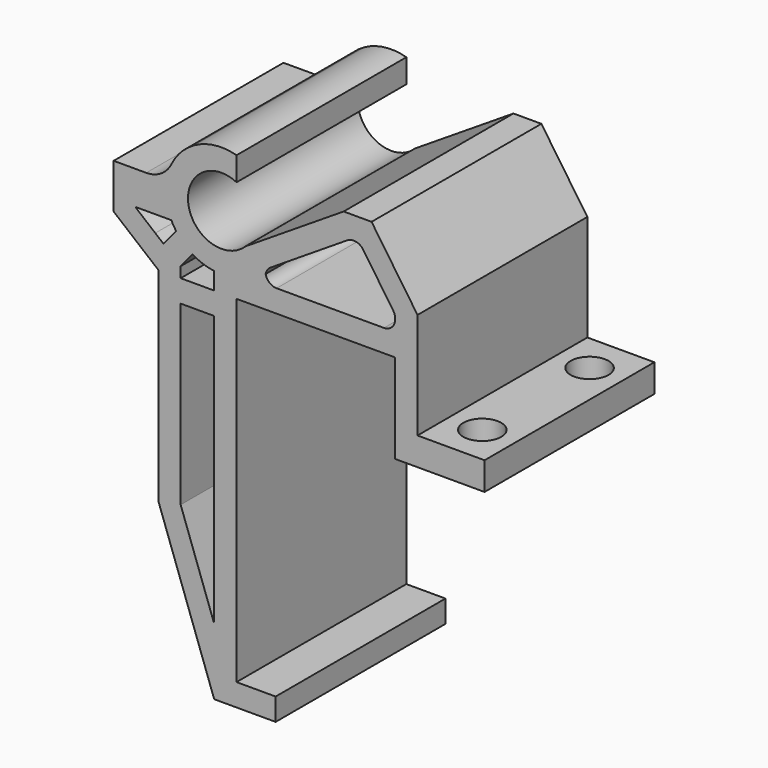
from build123d import *

# Parameters (mm, degrees)
F0_W        = 3
F0_H        = 2
F1_DEPTH    = 19
F3_D        = 3.4
F4_T1_DEPTH = 19


# Not quite as in the source:
# - a fillet or chamfer that OpenCascade refuses, or shapes differently, is made with other operations: its cross-section is extruded or revolved along the edge and cut away or added


with BuildPart() as f1:
    # F0 (on Front) → F1 (new body)
    with BuildSketch(Plane.XZ):
        with Locations((-7, 31.2)):
            Rectangle(F0_W, F0_H)
        with BuildLine():
            Line((-10.0427465571, 34.4155443421), (-8.5, 33.1427784325))
            Line((-8.5, 33.1427784325), (-7.441074238, 34.4263248107))
            ThreePointArc((-7.441074238, 34.4263248107), (-8.244619139, 35.032889635), (-8.9103596286, 35.7881345584))
            Line((-8.9103596286, 35.7881345584), (-10.0427465571, 34.4155443421))
        make_face()
        with BuildLine():
            Line((-10.5, 14), (-5.5, 0))
            Line((-5.5, 0), (-5.5, 5.9464274989))
            Line((-5.5, 5.9464274989), (-8.5, 14.3464274989))
            Line((-8.5, 14.3464274989), (-8.5, 30.2))
            Line((-8.5, 30.2), (-8.5, 32.2))
            Line((-8.5, 32.2), (-8.5, 33.1427784325))
            Line((-8.5, 33.1427784325), (-10.0427465571, 34.4155443421))
            Line((-10.0427465571, 34.4155443421), (-10.7699806475, 35.0155124667))
            Line((-10.7699806475, 35.0155124667), (-12.5, 36.4427784325))
            Line((-12.5, 36.4427784325), (-12.5, 36.5))
            Line((-12.5, 36.5), (-9.3357403136, 36.5))
            ThreePointArc((-9.3357403136, 36.5), (-9.7907115521, 37.9601557031), (-9.7830217401, 39.4895328221))
            ThreePointArc((-9.7830217401, 39.4895328221), (-9.7333018776, 39.7544433664), (-9.6693788597, 40.0162897125))
            ThreePointArc((-9.6693788597, 40.0162897125), (-9.5234750406, 40.4660413374), (-9.3357403136, 40.9))
            ThreePointArc((-9.3357403136, 40.9), (-10.2578590901, 39.8786796564), (-11.5807347457, 39.5))
            Line((-11.5807347457, 39.5), (-14.5, 39.5))
            Line((-14.5, 39.5), (-14.5, 35.5))
            Line((-14.5, 35.5), (-10.5, 32.2))
            Line((-10.5, 32.2), (-10.5, 14))
        make_face()
        with BuildLine():
            Line((-4.3254974298, 0), (0, 0))
            Line((0, 0), (0, 2))
            Line((0, 2), (-3.5, 2))
            Line((-3.5, 2), (-3.5, 32.2))
            Line((-3.5, 32.2), (6, 32.2))
            Line((6, 32.2), (10.7, 32.2))
            Line((10.7, 32.2), (10.7, 24.2))
            Line((10.7, 24.2), (18.7, 24.2))
            Line((18.7, 24.2), (18.7, 26.7))
            Line((18.7, 26.7), (12.7, 26.7))
            Line((12.7, 26.7), (12.7, 36.2))
            Line((12.7, 36.2), (8.5871078054, 42.2))
            Line((8.5871078054, 42.2), (6.0871078054, 42.2))
            Line((6.0871078054, 42.2), (6, 42.14441707))
            Line((6, 42.14441707), (-2.7279451008, 36.5751714729))
            ThreePointArc((-2.7279451008, 36.5751714729), (-2.80839002, 36.4979195279), (-2.8916508552, 36.4237111635))
            ThreePointArc((-2.8916508552, 36.4237111635), (-7.1777694161, 36.8127553939), (-6.6645515402, 41.085784196))
            ThreePointArc((-6.6645515402, 41.085784196), (-6.4594906698, 41.2290009349), (-6.2432123403, 41.3546380278))
            ThreePointArc((-6.2432123403, 41.3546380278), (-4.8748228701, 41.6998591388), (-3.5, 41.3812223027))
            Line((-3.5, 41.3812223027), (-3.5, 43.5154909445))
            ThreePointArc((-3.5, 43.5154909445), (-5.4216118426, 43.6667277767), (-7.2576401277, 43.0798165491))
            Line((-7.2576401277, 43.0798165491), (-7.8017760466, 42.7326069212))
            ThreePointArc((-7.8017760466, 42.7326069212), (-8.6798603613, 41.909300368), (-9.3357403136, 40.9))
            ThreePointArc((-9.3357403136, 40.9), (-9.5234750406, 40.4660413374), (-9.6693788597, 40.0162897125))
            ThreePointArc((-9.6693788597, 40.0162897125), (-9.7333018776, 39.7544433664), (-9.7830217401, 39.4895328221))
            ThreePointArc((-9.7830217401, 39.4895328221), (-9.7907115521, 37.9601557031), (-9.3357403136, 36.5))
            ThreePointArc((-9.3357403136, 36.5), (-9.1378337815, 36.1352330993), (-8.9103596286, 35.7881345584))
            ThreePointArc((-8.9103596286, 35.7881345584), (-8.244619139, 35.032889635), (-7.441074238, 34.4263248107))
            ThreePointArc((-7.441074238, 34.4263248107), (-6.506072339, 33.9837160238), (-5.5, 33.7429889213))
            Line((-5.5, 33.7429889213), (-5.5, 32.3898009956))
            Line((-5.5, 32.3898009956), (-5.5, 32.2))
            Line((-5.5, 32.2), (-5.5, 30.2))
            Line((-5.5, 30.2), (-5.5, 5.9464274989))
            Line((-5.5, 5.9464274989), (-5.5, 0))
            Line((-5.5, 0), (-4.3254974298, 0))
        make_face()
        Polygon((-0.9128921946, 34.2), (-0.9128921946, 35.3608666872), (6.6708440859, 40.2), (7.5332950832, 40.2), (10.7, 35.5803239662), (10.7, 34.2), align=None, mode=Mode.SUBTRACT)
    extrude(amount=F1_DEPTH)

    # F3 (through all)
    with Locations(Plane.XY.offset(26.7)):
        with Locations((15.7, -15.5), (15.7, -3.5)):
            Hole(F3_D / 2)

    # F4: fillet of radius 1 on 6 edges, made by hand

    # F4_s2 → F4_t1 (join)
    with BuildSketch(Plane.XZ):
        with BuildLine():
            ThreePointArc((10.5248181897, 35.8358839984), (10.6552010756, 35.5664435563), (10.7, 35.2704859494))
            Line((10.7, 35.2704859494), (10.7, 35.5803239662))
            Line((10.7, 35.5803239662), (10.5248181897, 35.8358839984))
        make_face()
        with BuildLine():
            ThreePointArc((7.0063887221, 40.2), (7.4725442492, 40.0847027888), (7.8312069118, 39.7653980491))
            Line((7.8312069118, 39.7653980491), (7.5332950832, 40.2))
            Line((7.5332950832, 40.2), (7.0063887221, 40.2))
        make_face()
        with BuildLine():
            ThreePointArc((6.4247991527, 40.0430003116), (6.6825339897, 40.1599479964), (6.9627122262, 40.2))
            Line((6.9627122262, 40.2), (6.6708440859, 40.2))
            Line((6.6708440859, 40.2), (6.4247991527, 40.0430003116))
        make_face()
        with BuildLine():
            ThreePointArc((-0.9128921946, 34.8127210695), (-0.7897938633, 35.2933908764), (-0.450805268, 35.6557213811))
            Line((-0.450805268, 35.6557213811), (-0.9128921946, 35.3608666872))
            Line((-0.9128921946, 35.3608666872), (-0.9128921946, 34.8127210695))
        make_face()
        with BuildLine():
            ThreePointArc((0.0871078054, 34.2), (-0.6199989757, 34.4928932188), (-0.9128921946, 35.2))
            Line((-0.9128921946, 35.2), (-0.9128921946, 34.2))
            Line((-0.9128921946, 34.2), (0.0871078054, 34.2))
        make_face()
        with BuildLine():
            ThreePointArc((9.7, 34.2), (10.4071067812, 34.4928932188), (10.7, 35.2))
            Line((10.7, 35.2), (10.7, 34.2))
            Line((10.7, 34.2), (9.7, 34.2))
        make_face()
    extrude(amount=F4_T1_DEPTH)


solid = f1.part
